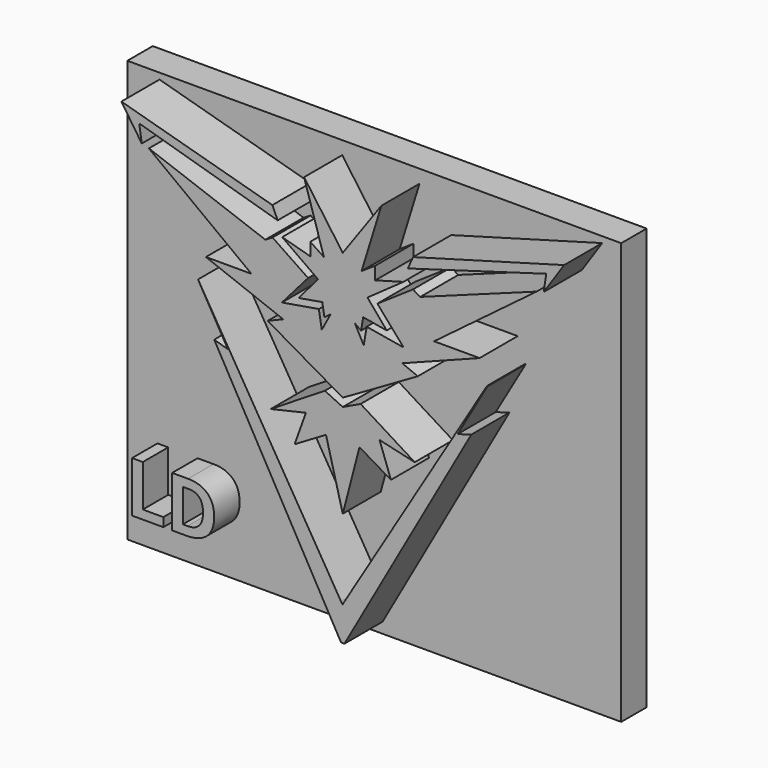
from build123d import *

# Parameters (mm, degrees)
F1_DEPTH     = 7.62
F2_W         = 78.9942257106
F2_H         = 67.4111880362
F3_DEPTH     = 5.08
F4_TEXT_SIZE = 11.3547604997
F5_DEPTH     = 5.08
F6_DEPTH     = 2.54


# Not quite as in the source:
# - Text() gives the source's letters only with a copy of the font that has no kerning and outlines rounded to 1/6400 em; it was checked with that copy


with BuildPart() as f1:
    # F0 (on Front) → F1 (new body)
    with BuildSketch(Plane.XZ):
        Polygon((11.9129230734, 36.592964083), (34.0614614543, 43.0456548929), (33.6538197007, 40.3485000134), (36.9149537291, 45.1965518296), (12.7621775027, 38.4707301855), align=None)
    extrude(amount=F1_DEPTH)


with BuildPart() as f1b:
    # F0 (on Front) → F1, piece 2 (new body)
    with BuildSketch(Plane.XZ):
        Polygon((1.2365910225, -13.7706054375), (-21.6437820345, 24.1314768791), (-16.8620757759, 15.8582236618), (-19.0530697121, 16.4965414683), (1.2357736705, -19.5464268327), (1.7781219212, -19.5464268327), (22.0669653039, 16.4965414683), (19.8759713676, 15.8582236618), (24.6576776262, 24.1314768791), (24.5885416961, 24.1776026134), (1.7081686392, -13.7244797032), (1.4697087634, -14.1567725591), align=None)
    extrude(amount=F1_DEPTH)


with BuildPart() as f1c:
    # F0 (on Front) → F1, piece 3 (new body)
    with BuildSketch(Plane.XZ):
        Polygon((1.5069477959, 13.6944502592), (-1.3545840047, 15.056328848), (-10.0100776181, 9.6693439409), (-4.3809800409, 10.9706940129), (-6.1968178488, 5.9468755499), (-1.1730002007, 8.9127449319), (1.5069477959, -1.3326546177), (4.1868957924, 8.9127449319), (9.2107134406, 5.9468755499), (7.3948756326, 10.9706940129), (13.0239732098, 9.6693439409), (4.3684795965, 15.056328848), align=None)
    extrude(amount=F1_DEPTH)


with BuildPart() as f1d:
    # F0 (on Front) → F1, piece 4 (new body)
    with BuildSketch(Plane.XZ):
        Polygon((-9.748281911, 38.4707301855), (-33.9010581374, 45.1965518296), (-30.639924109, 40.3485000134), (-31.0475658625, 43.0456548929), (-8.8990274817, 36.592964083), align=None)
    extrude(amount=F1_DEPTH)


with BuildPart() as f1e:
    # F0 (on Front) → F1, piece 5 (new body)
    with BuildSketch(Plane.XZ):
        Polygon((7.6874790248, 44.0543666482), (1.5069477959, 35.4088284075), (-4.673583433, 44.0543666482), (-1.5064048348, 33.825237304), (-3.6891899072, 35.2804288268), (-3.6891899072, 33.2260429859), (-8.1831589341, 34.4672352076), (-2.447998384, 30.4012615234), (-5.5295773782, 26.7632864416), (-1.7632032977, 27.4052824825), (-1.421541232, 25.4008664631), (-0.4364121996, 26.1212904006), (-1.8488025526, 23.467708379), (-2.3195990361, 26.2496899813), (-8.2234673373, 25.2505746625), (-4.0315873921, 30.0588645041), (-9.7239483148, 33.9108370245), (-10.8795408159, 33.2260429859), (-29.4974129647, 40.0311946869), (-13.1051251665, 27.7048796415), (-20.3810762614, 27.7048796415), (-8.0119594932, 22.9541100562), (-10.4943430051, 21.9269189984), (1.5069477959, 15.0113655254), (13.5082385968, 21.9269189984), (11.0258550849, 22.9541100562), (23.3949718531, 27.7048796415), (16.1190207582, 27.7048796415), (32.5113085564, 40.0311946869), (13.8934364077, 33.2260429859), (12.7378439065, 33.9108370245), (7.0454829838, 30.0588645041), (11.2373629291, 25.2505746625), (5.3334946278, 26.2496899813), (4.8626981443, 23.467708379), (3.4503077914, 26.1212904006), (4.4354368237, 25.4008664631), (4.7770988895, 27.4052824825), (8.5434729699, 26.7632864416), (5.4618939757, 30.4012615234), (11.1970545258, 34.4672352076), (6.7030854989, 33.2260429859), (6.7030854989, 35.2804288268), (4.5203004265, 33.825237304), align=None)
    extrude(amount=F1_DEPTH)


with BuildPart() as f3:
    # F2 (on face) → F3 (new body)
    with BuildSketch(Plane(origin=(0, 0, 0), x_dir=(-1, 0, 0), z_dir=(0, 1, 0))):
        with Locations((-0.4544910043, 12.464730069)):
            Rectangle(F2_W, F2_H)
    extrude(amount=F3_DEPTH)

    # F4 (on face) → F5 (join)
    with BuildSketch(Plane.XZ):
        with Locations((-35.2478586137, -14.2509592697)):
            Text('LD', F4_TEXT_SIZE, font='Open Sans', font_style=FontStyle.BOLD, text_align=(TextAlign.LEFT, TextAlign.BOTTOM))
    extrude(amount=F5_DEPTH)

    # F4 (on face) → F6 (join)
    with BuildSketch(Plane.XZ):
        with Locations((-35.2478586137, -14.2509592697)):
            Text('LD', F4_TEXT_SIZE, font='Open Sans', font_style=FontStyle.BOLD, text_align=(TextAlign.LEFT, TextAlign.BOTTOM))
    extrude(amount=F6_DEPTH)


solid = Compound([f1.part, f1b.part, f1c.part, f1d.part, f1e.part, f3.part])
